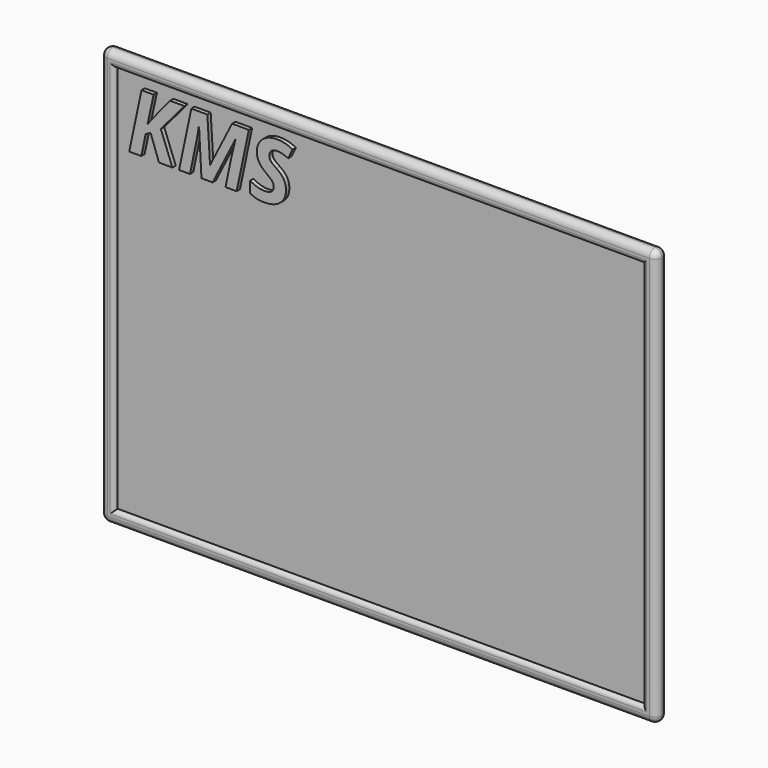
from build123d import *

# Parameters (mm, degrees)
F0_W          = 400
F0_H          = 300
F0_W_2        = 380
F0_H_2        = 280
F1_DEPTH      = 10
F2_DEPTH      = 7
F3_R          = 2.99999
F4_R          = 2.99999
F5_R          = 2.99999
F6_R          = 2.99999
F7_R          = 5
F8_R          = 5
F9_R          = 4.99999
F10_TEXT_SIZE = 58.5014621417
F11_DEPTH     = 3
F12_R         = 50
F13_DEPTH     = 2
F14_R         = 25
F15_DEPTH     = 2
F16_R         = 10
F17_DEPTH     = 2
F18_R         = 4.5
F19_DEPTH     = 2
F20_R         = 1.5
F21_DEPTH     = 7


# Not quite as in the source:
# - a fillet or chamfer is up to 0.001 mm smaller than in the source, because OpenCascade refuses the exact size
# - Text() gives the source's letters only with a copy of the font that has no kerning and outlines rounded to 1/6400 em; it was checked with that copy


with BuildPart() as f1:
    # F0 (on Front) → F1 (new body)
    with BuildSketch(Plane.XZ):
        with Locations((124.9697551131, 109.8084688187)):
            Rectangle(F0_W, F0_H)
        with Locations((124.9697551131, 109.8084688187)):
            Rectangle(F0_W_2, F0_H_2, mode=Mode.SUBTRACT)
    extrude(amount=F1_DEPTH)

    # F0 (on Front) → F2 (join)
    with BuildSketch(Plane.XZ):
        with Locations((124.9697551131, 109.8084688187)):
            Rectangle(F0_W_2, F0_H_2)
    extrude(amount=F2_DEPTH)

    # F3 (radius 3 in the source; OpenCascade refuses exactly that, so slightly less here)
    f3_edges = [f1.edges().sort_by_distance(p)[0] for p in [
        (-65.030245, -10, 109.808469),
    ]]
    fillet(f3_edges, radius=F3_R)

    # F4 (radius 3 in the source; OpenCascade refuses exactly that, so slightly less here)
    f4_edges = [f1.edges().sort_by_distance(p)[0] for p in [
        (314.969755, -10, 109.808469),
    ]]
    fillet(f4_edges, radius=F4_R)

    # F5 (radius 3 in the source; OpenCascade refuses exactly that, so slightly less here)
    f5_edges = [f1.edges().sort_by_distance(p)[0] for p in [
        (124.969755, -10, -30.191531),
    ]]
    fillet(f5_edges, radius=F5_R)

    # F6 (radius 3 in the source; OpenCascade refuses exactly that, so slightly less here)
    f6_edges = [f1.edges().sort_by_distance(p)[0] for p in [
        (124.969755, -10, 249.808469),
    ]]
    fillet(f6_edges, radius=F6_R)

    # F7
    f7_edges = [f1.edges().sort_by_distance(p)[0] for p in [
        (324.969755, -5, 259.808469),
        (324.969755, -5, -40.191531),
        (-75.030245, -5, -40.191531),
        (-75.030245, -5, 259.808469),
    ]]
    fillet(f7_edges, radius=F7_R)

    # F8
    f8_edges = [f1.edges().sort_by_distance(p)[0] for p in [
        (-75.030245, -10, 109.808469),
    ]]
    fillet(f8_edges, radius=F8_R)

    # F9 (radius 5 in the source; OpenCascade refuses exactly that, so slightly less here)
    f9_edges = [f1.edges().sort_by_distance(p)[0] for p in [
        (-75.030245, 0, 109.808469),
    ]]
    fillet(f9_edges, radius=F9_R)

    # F10 (on face) → F11 (join)
    with BuildSketch(Plane.XZ.offset(7)):
        with Locations((-55.8700188994, 200.7444947958)):
            Text('KMS', F10_TEXT_SIZE, font='Open Sans', font_style=FontStyle.BOLDITALIC, text_align=(TextAlign.LEFT, TextAlign.BOTTOM))
    extrude(amount=F11_DEPTH)

    # F12 (on face) → F13 (join)
    with BuildSketch(Plane.XZ):
        with Locations((124.9691992998, 109.8101139069)):
            Circle(F12_R)
    extrude(amount=-F13_DEPTH)

    # F14 (on face) → F15 (join)
    with BuildSketch(Plane(origin=(0, 2, 0), x_dir=(-1, 0, 0), z_dir=(0, 1, 0))):
        with Locations((-124.9691992998, 109.8101139069)):
            Circle(F14_R)
    extrude(amount=F15_DEPTH)

    # F16 (on face) → F17 (join)
    with BuildSketch(Plane(origin=(0, 4, 0), x_dir=(-1, 0, 0), z_dir=(0, 1, 0))):
        with Locations((-124.9691992998, 109.8101139069)):
            Circle(F16_R)
    extrude(amount=F17_DEPTH)

    # F18 (on face) → F19 (join)
    with BuildSketch(Plane(origin=(0, 6, 0), x_dir=(-1, 0, 0), z_dir=(0, 1, 0))):
        with Locations((-124.9691992998, 109.8101139069)):
            Circle(F18_R)
    extrude(amount=F19_DEPTH)

    # F20 (on face) → F21 (cut)
    with BuildSketch(Plane(origin=(0, 8, 0), x_dir=(-1, 0, 0), z_dir=(0, 1, 0))):
        with Locations((-124.9691992998, 109.8101139069)):
            Circle(F20_R)
    extrude(amount=-F21_DEPTH, mode=Mode.SUBTRACT)


solid = f1.part
